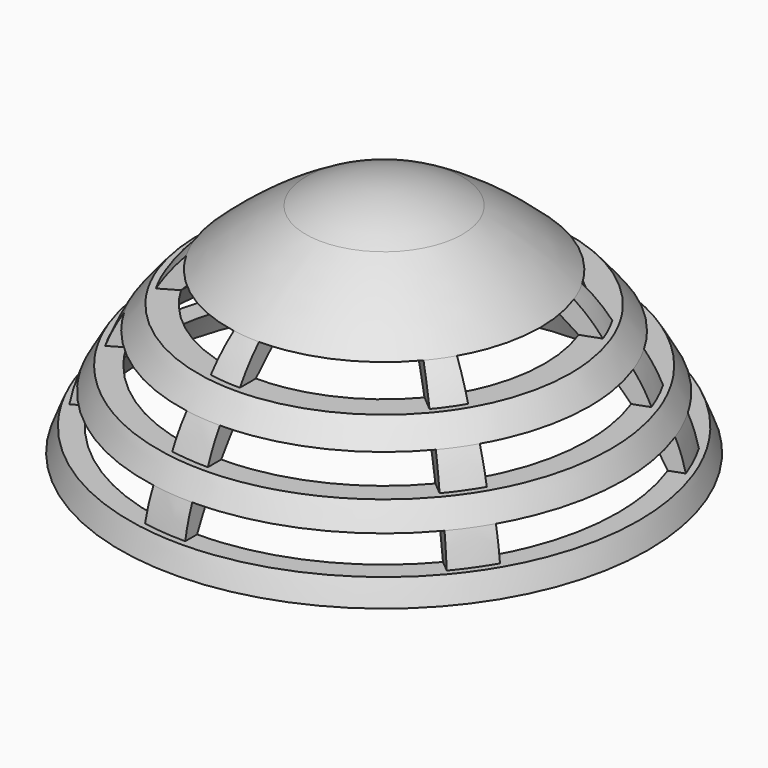
from build123d import *

# Parameters (mm, degrees)
F3_T             = -12.5
F5_DEPTH         = 20
F5_COPIES_COUNT  = 6
F8_DEPTH         = 20
F8_COPIES_COUNT  = 6
F11_DEPTH        = 20
F11_COPIES_COUNT = 6


# Not quite as in the source:
# - a pattern or mirror of a feature is missing from the dataset's text; its kind, count and spacing are read off the source's solid


with BuildPart() as f1:
    # F0 (on Front) → F1 (revolve)
    with BuildSketch(Plane.XZ):
        with BuildLine():
            Line((0, 155), (0, 0))
            Line((0, 0), (172.1073224064, 0))
            ThreePointArc((172.1073224064, 0), (124.3329517712, 81.8069606221), (51, 141.7823512447))
            ThreePointArc((51, 141.7823512447), (26.3424858291, 151.6418882171), (0, 155))
        make_face()
    revolve(axis=Axis((0, 0, 77.5), (0, 0, 1)))

    # F3
    f3_openings = [f1.faces().sort_by_distance(p)[0] for p in [
        (0, 0, 0),
    ]]
    offset(amount=F3_T, openings=f3_openings)

    # F4 (on offset) → F5 (cut)
    with BuildSketch(Plane.XY.offset(35)):
        with BuildLine():
            Line((141.718221977, -118.915707792), (0, 0))
            Line((0, 0), (0, -185))
            ThreePointArc((0, -185), (78.184378422, -167.6669406018), (141.718221977, -118.915707792))
        make_face()
    f5 = extrude(amount=-F5_DEPTH, mode=Mode.SUBTRACT)

    # F5_copies: F5 ×6 about axis
    f5_copies_axis = Axis((0, 0, 0), (0, 0, 1))
    for i in range(1, F5_COPIES_COUNT):
        add(f5.rotate(f5_copies_axis, i * 360 / F5_COPIES_COUNT), mode=Mode.SUBTRACT)

    # F7 (on offset) → F8 (cut)
    with BuildSketch(Plane.XY.offset(70)):
        with BuildLine():
            Line((141.718221977, -118.915707792), (0, 0))
            Line((0, 0), (0, -185))
            ThreePointArc((0, -185), (78.184378422, -167.6669406018), (141.718221977, -118.915707792))
        make_face()
    f8 = extrude(amount=-F8_DEPTH, mode=Mode.SUBTRACT)

    # F8_copies: F8 ×6 about axis
    f8_copies_axis = Axis((0, 0, 0), (0, 0, 1))
    for i in range(1, F8_COPIES_COUNT):
        add(f8.rotate(f8_copies_axis, i * 360 / F8_COPIES_COUNT), mode=Mode.SUBTRACT)

    # F10 (on offset) → F11 (cut)
    with BuildSketch(Plane.XY.offset(105)):
        with BuildLine():
            Line((141.718221977, -118.915707792), (0, 0))
            Line((0, 0), (0, -185))
            ThreePointArc((0, -185), (78.184378422, -167.6669406018), (141.718221977, -118.915707792))
        make_face()
    f11 = extrude(amount=-F11_DEPTH, mode=Mode.SUBTRACT)

    # F11_copies: F11 ×6 about axis
    f11_copies_axis = Axis((0, 0, 0), (0, 0, 1))
    for i in range(1, F11_COPIES_COUNT):
        add(f11.rotate(f11_copies_axis, i * 360 / F11_COPIES_COUNT), mode=Mode.SUBTRACT)

    # F12 (on Right) → F13 (revolve, cut)
    with BuildSketch(Plane.YZ):
        with BuildLine():
            ThreePointArc((-101.9649581459, 105), (-77.5685770824, 124.8960533075), (-51, 141.7823512447))
            ThreePointArc((-51, 141.7823512447), (-26.3424858291, 151.6418882171), (0, 155))
            Line((0, 155), (0, 185))
            Line((0, 185), (-197.1073224064, 185))
            Line((-197.1073224064, 185), (-197.1073224064, 0))
            Line((-197.1073224064, 0), (-172.1073224064, 0))
            ThreePointArc((-172.1073224064, 0), (-169.2211094959, 7.5453856323), (-166.1079448786, 15))
            Line((-166.1079448786, 15), (-162.1079448786, 15))
            ThreePointArc((-162.1079448786, 15), (-159.7444782713, 25.1419985247), (-156.3880046172, 35))
            ThreePointArc((-156.3880046172, 35), (-152.1503575715, 42.5708403698), (-147.668966763, 50))
            Line((-147.668966763, 50), (-143.668966763, 50))
            ThreePointArc((-143.668966763, 50), (-139.2923081775, 60.2611225001), (-133.8517162634, 70))
            ThreePointArc((-133.8517162634, 70), (-127.8428338637, 77.6116153385), (-121.5615021699, 85))
            Line((-121.5615021699, 85), (-117.5615021699, 85))
            ThreePointArc((-117.5615021699, 85), (-110.369315466, 95.4726418095), (-101.9649581459, 105))
        make_face()
    revolve(axis=Axis((0, 0, 77.5), (0, 0, 1)), mode=Mode.SUBTRACT)


solid = f1.part
